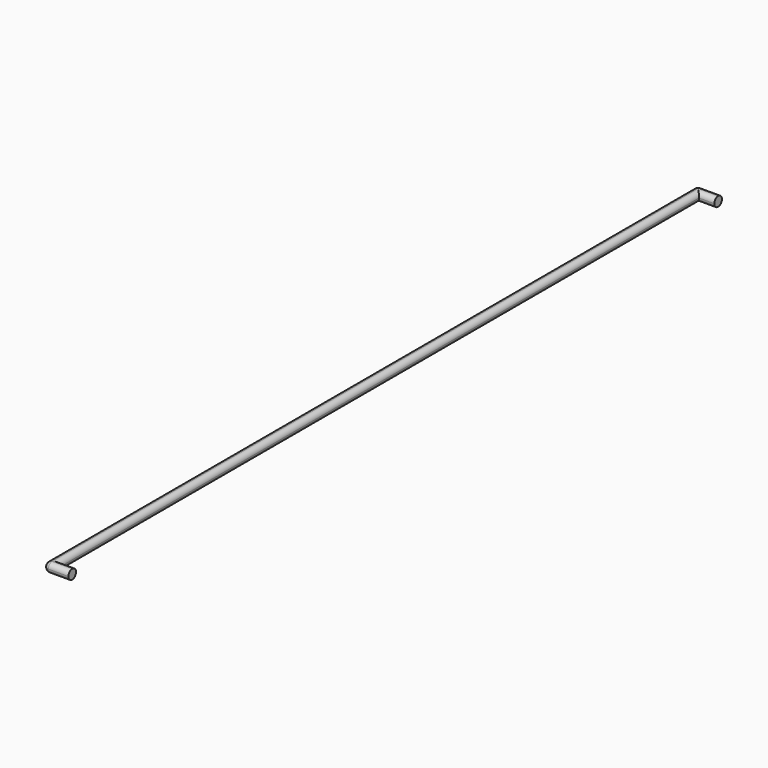
from build123d import *

# Parameters (mm, degrees)
F0_W     = 3.9624
F0_H     = 3.9624
F1_DEPTH = 339.725
F2_W     = 3.9624
F2_H     = 3.9624
F3_DEPTH = 6.35
F4_R     = 1.98119


# Not quite as in the source:
# - a fillet or chamfer is up to 0.001 mm smaller than in the source, because OpenCascade refuses the exact size


with BuildPart() as f1:
    # F0 (on Front) → F1 (new body)
    with BuildSketch(Plane.XZ):
        Rectangle(F0_W, F0_H)
    extrude(amount=F1_DEPTH)

    # F2 (on face) → F3 (join)
    with BuildSketch(Plane.YZ.offset(1.9812)):
        with Locations((-337.7438, 0)):
            Rectangle(F2_W, F2_H)
        with Locations((-1.9812, 0)):
            Rectangle(F2_W, F2_H)
    extrude(amount=F3_DEPTH)

    # F4 (radius 1.9812 in the source; OpenCascade refuses exactly that, so slightly less here)
    f4_edges = [f1.edges().sort_by_distance(p)[0] for p in [
        (3.175, 0, 1.9812),
        (3.175, 0, -1.9812),
        (-1.9812, -169.8625, 1.9812),
        (1.9812, -169.8625, 1.9812),
        (-1.9812, -169.8625, -1.9812),
        (1.9812, -169.8625, -1.9812),
        (-1.9812, 0, 0),
        (3.175, -339.725, 1.9812),
        (3.175, -339.725, -1.9812),
        (-1.9812, -339.725, 0),
        (5.1562, -335.7626, -1.9812),
        (5.1562, -3.9624, -1.9812),
        (5.1562, -335.7626, 1.9812),
        (5.1562, -3.9624, 1.9812),
    ]]
    fillet(f4_edges, radius=F4_R)


solid = f1.part
